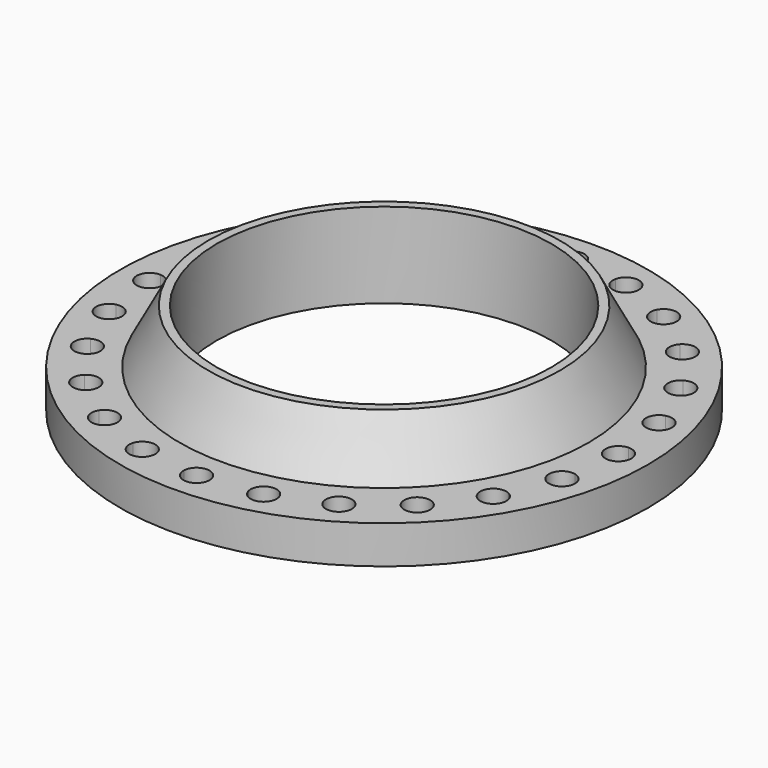
from build123d import *

# Parameters (mm, degrees)
F0_R     = 45.75
F0_R_2   = 35.5
F0_R_3   = 29
F1_DEPTH = 6.6
F3_DEPTH = 16
F5_R     = 34.75
F6_DEPTH = 1.25


# Not quite as in the source:
# - a fillet or chamfer that OpenCascade refuses, or shapes differently, is made with other operations: its cross-section is extruded or revolved along the edge and cut away or added
# - the program builds the solid bodies; features that only make, move or delete a surface that nothing else refers to are left out


with BuildPart() as f1:
    # F0 (on Top) → F1 (new body)
    with BuildSketch(Plane.XY):
        Circle(F0_R)
        with BuildLine():
            ThreePointArc((39.7626716036, 8.3258976659), (40.2774474933, 5.3026265589), (40.5626923077, 2.2491371126))
            ThreePointArc((40.5626923077, 2.2491371126), (42.1938065037, 1.6128689202), (42.875, 0))
            ThreePointArc((42.875, 0), (42.1938065037, -1.6128689202), (40.5626923077, -2.2491371126))
            ThreePointArc((40.5626923077, -2.2491371126), (40.2774474933, -5.3026265589), (39.7626716036, -8.3258976659))
            ThreePointArc((39.7626716036, -8.3258976659), (41.0066434783, -9.1202234435), (41.490736693, -10.5145237073))
            ThreePointArc((41.490736693, -10.5145237073), (40.5856002009, -12.3183646496), (38.598432564, -12.6708969138))
            ThreePointArc((38.598432564, -12.6708969138), (37.5326060083, -15.5465144398), (36.2528905407, -18.3335362777))
            ThreePointArc((36.2528905407, -18.3335362777), (37.115073941, -19.1606252568), (37.4322820287, -20.3125))
            ThreePointArc((37.4322820287, -20.3125), (36.2801915533, -22.2764487457), (34.003753428, -22.22915603))
            ThreePointArc((34.003753428, -22.22915603), (32.2299794493, -24.7309330535), (30.2725348981, -27.0917746898))
            ThreePointArc((30.2725348981, -27.0917746898), (30.7928194193, -27.8364726592), (30.9762129857, -28.7262129857))
            ThreePointArc((30.9762129857, -28.7262129857), (29.5583829906, -30.8166658273), (27.0917746898, -30.2725348981))
            ThreePointArc((27.0917746898, -30.2725348981), (24.7309330535, -32.2299794493), (22.22915603, -34.003753428))
            ThreePointArc((22.22915603, -34.003753428), (22.477560746, -34.5698998227), (22.5625, -35.1822820287))
            ThreePointArc((22.5625, -35.1822820287), (20.8646918257, -37.3634707385), (18.3335362777, -36.2528905407))
            ThreePointArc((18.3335362777, -36.2528905407), (15.5465144398, -37.5326060083), (12.6708969138, -38.598432564))
            ThreePointArc((12.6708969138, -38.598432564), (12.740993976, -38.9161906367), (12.7645237073, -39.240736693))
            ThreePointArc((12.7645237073, -39.240736693), (10.7772891986, -41.4753405274), (8.3258976659, -39.7626716036))
            ThreePointArc((8.3258976659, -39.7626716036), (5.3026265589, -40.2774474933), (2.2491371126, -40.5626923077))
            ThreePointArc((2.2491371126, -40.5626923077), (2.2497842678, -40.5938431665), (2.25, -40.625))
            ThreePointArc((2.25, -40.625), (-0.0311568335, -42.8747842678), (-2.2491371126, -40.5626923077))
            ThreePointArc((-2.2491371126, -40.5626923077), (-5.3026265589, -40.2774474933), (-8.3258976659, -39.7626716036))
            ThreePointArc((-8.3258976659, -39.7626716036), (-11.0968665588, -41.4140698021), (-12.6708969138, -38.598432564))
            ThreePointArc((-12.6708969138, -38.598432564), (-15.5465144398, -37.5326060083), (-18.3335362777, -36.2528905407))
            ThreePointArc((-18.3335362777, -36.2528905407), (-21.4375, -37.1308391873), (-22.22915603, -34.003753428))
            ThreePointArc((-22.22915603, -34.003753428), (-24.7309330535, -32.2299794493), (-27.0917746898, -30.2725348981))
            ThreePointArc((-27.0917746898, -30.2725348981), (-30.3172032434, -30.3172032434), (-30.2725348981, -27.0917746898))
            ThreePointArc((-30.2725348981, -27.0917746898), (-32.2299794493, -24.7309330535), (-34.003753428, -22.22915603))
            ThreePointArc((-34.003753428, -22.22915603), (-37.1308391873, -21.4375), (-36.2528905407, -18.3335362777))
            ThreePointArc((-36.2528905407, -18.3335362777), (-37.5326060083, -15.5465144398), (-38.598432564, -12.6708969138))
            ThreePointArc((-38.598432564, -12.6708969138), (-41.4140698021, -11.0968665588), (-39.7626716036, -8.3258976659))
            ThreePointArc((-39.7626716036, -8.3258976659), (-40.2774474933, -5.3026265589), (-40.5626923077, -2.2491371126))
            ThreePointArc((-40.5626923077, -2.2491371126), (-42.875, 0), (-40.5626923077, 2.2491371126))
            ThreePointArc((-40.5626923077, 2.2491371126), (-40.2774474933, 5.3026265589), (-39.7626716036, 8.3258976659))
            ThreePointArc((-39.7626716036, 8.3258976659), (-41.4140698021, 11.0968665588), (-38.598432564, 12.6708969138))
            ThreePointArc((-38.598432564, 12.6708969138), (-37.5326060083, 15.5465144398), (-36.2528905407, 18.3335362777))
            ThreePointArc((-36.2528905407, 18.3335362777), (-37.1308391873, 21.4375), (-34.003753428, 22.22915603))
            ThreePointArc((-34.003753428, 22.22915603), (-32.2299794493, 24.7309330535), (-30.2725348981, 27.0917746898))
            ThreePointArc((-30.2725348981, 27.0917746898), (-30.3172032434, 30.3172032434), (-27.0917746898, 30.2725348981))
            ThreePointArc((-27.0917746898, 30.2725348981), (-24.7309330535, 32.2299794493), (-22.22915603, 34.003753428))
            ThreePointArc((-22.22915603, 34.003753428), (-21.4375, 37.1308391873), (-18.3335362777, 36.2528905407))
            ThreePointArc((-18.3335362777, 36.2528905407), (-15.5465144398, 37.5326060083), (-12.6708969138, 38.598432564))
            ThreePointArc((-12.6708969138, 38.598432564), (-11.0968665588, 41.4140698021), (-8.3258976659, 39.7626716036))
            ThreePointArc((-8.3258976659, 39.7626716036), (-5.3026265589, 40.2774474933), (-2.2491371126, 40.5626923077))
            ThreePointArc((-2.2491371126, 40.5626923077), (-0.0311568335, 42.8747842678), (2.25, 40.625))
            ThreePointArc((2.25, 40.625), (2.2497842678, 40.5938431665), (2.2491371126, 40.5626923077))
            ThreePointArc((2.2491371126, 40.5626923077), (5.3026265589, 40.2774474933), (8.3258976659, 39.7626716036))
            ThreePointArc((8.3258976659, 39.7626716036), (10.7772891986, 41.4753405274), (12.7645237073, 39.240736693))
            ThreePointArc((12.7645237073, 39.240736693), (12.740993976, 38.9161906367), (12.6708969138, 38.598432564))
            ThreePointArc((12.6708969138, 38.598432564), (15.5465144398, 37.5326060083), (18.3335362777, 36.2528905407))
            ThreePointArc((18.3335362777, 36.2528905407), (20.8646918257, 37.3634707385), (22.5625, 35.1822820287))
            ThreePointArc((22.5625, 35.1822820287), (22.477560746, 34.5698998227), (22.22915603, 34.003753428))
            ThreePointArc((22.22915603, 34.003753428), (24.7309330535, 32.2299794493), (27.0917746898, 30.2725348981))
            ThreePointArc((27.0917746898, 30.2725348981), (29.5583829906, 30.8166658273), (30.9762129857, 28.7262129857))
            ThreePointArc((30.9762129857, 28.7262129857), (30.7928194193, 27.8364726592), (30.2725348981, 27.0917746898))
            ThreePointArc((30.2725348981, 27.0917746898), (32.2299794493, 24.7309330535), (34.003753428, 22.22915603))
            ThreePointArc((34.003753428, 22.22915603), (36.2801915533, 22.2764487457), (37.4322820287, 20.3125))
            ThreePointArc((37.4322820287, 20.3125), (37.115073941, 19.1606252568), (36.2528905407, 18.3335362777))
            ThreePointArc((36.2528905407, 18.3335362777), (37.5326060083, 15.5465144398), (38.598432564, 12.6708969138))
            ThreePointArc((38.598432564, 12.6708969138), (40.5856002009, 12.3183646496), (41.490736693, 10.5145237073))
            ThreePointArc((41.490736693, 10.5145237073), (41.0066434783, 9.1202234435), (39.7626716036, 8.3258976659))
        make_face(mode=Mode.SUBTRACT)
        with BuildLine():
            ThreePointArc((40.5626923077, -2.2491371126), (38.375, 0), (40.5626923077, 2.2491371126))
            ThreePointArc((40.5626923077, 2.2491371126), (40.2774474933, 5.3026265589), (39.7626716036, 8.3258976659))
            ThreePointArc((39.7626716036, 8.3258976659), (37.0674035838, 9.9321808558), (38.598432564, 12.6708969138))
            ThreePointArc((38.598432564, 12.6708969138), (37.5326060083, 15.5465144398), (36.2528905407, 18.3335362777))
            ThreePointArc((36.2528905407, 18.3335362777), (33.2337248702, 19.1875), (34.003753428, 22.22915603))
            ThreePointArc((34.003753428, 22.22915603), (32.2299794493, 24.7309330535), (30.2725348981, 27.0917746898))
            ThreePointArc((30.2725348981, 27.0917746898), (27.135222728, 27.135222728), (27.0917746898, 30.2725348981))
            ThreePointArc((27.0917746898, 30.2725348981), (24.7309330535, 32.2299794493), (22.22915603, 34.003753428))
            ThreePointArc((22.22915603, 34.003753428), (19.1875, 33.2337248702), (18.3335362777, 36.2528905407))
            ThreePointArc((18.3335362777, 36.2528905407), (15.5465144398, 37.5326060083), (12.6708969138, 38.598432564))
            ThreePointArc((12.6708969138, 38.598432564), (9.9321808558, 37.0674035838), (8.3258976659, 39.7626716036))
            ThreePointArc((8.3258976659, 39.7626716036), (5.3026265589, 40.2774474933), (2.2491371126, 40.5626923077))
            ThreePointArc((2.2491371126, 40.5626923077), (0, 38.375), (-2.2491371126, 40.5626923077))
            ThreePointArc((-2.2491371126, 40.5626923077), (-5.3026265589, 40.2774474933), (-8.3258976659, 39.7626716036))
            ThreePointArc((-8.3258976659, 39.7626716036), (-8.2799198729, 39.5035021843), (-8.2645237073, 39.240736693))
            ThreePointArc((-8.2645237073, 39.240736693), (-10.189977651, 37.0142664243), (-12.6708969138, 38.598432564))
            ThreePointArc((-12.6708969138, 38.598432564), (-15.5465144398, 37.5326060083), (-18.3335362777, 36.2528905407))
            ThreePointArc((-18.3335362777, 36.2528905407), (-18.1313112902, 35.7344738545), (-18.0625, 35.1822820287))
            ThreePointArc((-18.0625, 35.1822820287), (-19.700117794, 33.0172212828), (-22.22915603, 34.003753428))
            ThreePointArc((-22.22915603, 34.003753428), (-24.7309330535, 32.2299794493), (-27.0917746898, 30.2725348981))
            ThreePointArc((-27.0917746898, 30.2725348981), (-26.6357601441, 29.5583829906), (-26.4762129857, 28.7262129857))
            ThreePointArc((-26.4762129857, 28.7262129857), (-27.8364726592, 26.6596065521), (-30.2725348981, 27.0917746898))
            ThreePointArc((-30.2725348981, 27.0917746898), (-32.2299794493, 24.7309330535), (-34.003753428, 22.22915603))
            ThreePointArc((-34.003753428, 22.22915603), (-33.218333283, 21.4104095246), (-32.9322820287, 20.3125))
            ThreePointArc((-32.9322820287, 20.3125), (-34.0304072855, 18.3797080878), (-36.2528905407, 18.3335362777))
            ThreePointArc((-36.2528905407, 18.3335362777), (-37.5326060083, 15.5465144398), (-38.598432564, 12.6708969138))
            ThreePointArc((-38.598432564, 12.6708969138), (-37.4368957507, 11.8593872152), (-36.990736693, 10.5145237073))
            ThreePointArc((-36.990736693, 10.5145237073), (-37.8464364292, 8.748616922), (-39.7626716036, 8.3258976659))
            ThreePointArc((-39.7626716036, 8.3258976659), (-40.2774474933, 5.3026265589), (-40.5626923077, 2.2491371126))
            ThreePointArc((-40.5626923077, 2.2491371126), (-39.0121310798, 1.5688065037), (-38.375, 0))
            ThreePointArc((-38.375, 0), (-39.0121310798, -1.5688065037), (-40.5626923077, -2.2491371126))
            ThreePointArc((-40.5626923077, -2.2491371126), (-40.2774474933, -5.3026265589), (-39.7626716036, -8.3258976659))
            ThreePointArc((-39.7626716036, -8.3258976659), (-37.8464364292, -8.748616922), (-36.990736693, -10.5145237073))
            ThreePointArc((-36.990736693, -10.5145237073), (-37.4368957507, -11.8593872152), (-38.598432564, -12.6708969138))
            ThreePointArc((-38.598432564, -12.6708969138), (-37.5326060083, -15.5465144398), (-36.2528905407, -18.3335362777))
            ThreePointArc((-36.2528905407, -18.3335362777), (-34.0304072855, -18.3797080878), (-32.9322820287, -20.3125))
            ThreePointArc((-32.9322820287, -20.3125), (-33.218333283, -21.4104095246), (-34.003753428, -22.22915603))
            ThreePointArc((-34.003753428, -22.22915603), (-32.2299794493, -24.7309330535), (-30.2725348981, -27.0917746898))
            ThreePointArc((-30.2725348981, -27.0917746898), (-27.8364726592, -26.6596065521), (-26.4762129857, -28.7262129857))
            ThreePointArc((-26.4762129857, -28.7262129857), (-26.6357601441, -29.5583829906), (-27.0917746898, -30.2725348981))
            ThreePointArc((-27.0917746898, -30.2725348981), (-24.7309330535, -32.2299794493), (-22.22915603, -34.003753428))
            ThreePointArc((-22.22915603, -34.003753428), (-19.700117794, -33.0172212828), (-18.0625, -35.1822820287))
            ThreePointArc((-18.0625, -35.1822820287), (-18.1313112902, -35.7344738545), (-18.3335362777, -36.2528905407))
            ThreePointArc((-18.3335362777, -36.2528905407), (-15.5465144398, -37.5326060083), (-12.6708969138, -38.598432564))
            ThreePointArc((-12.6708969138, -38.598432564), (-10.189977651, -37.0142664243), (-8.2645237073, -39.240736693))
            ThreePointArc((-8.2645237073, -39.240736693), (-8.2799198729, -39.5035021843), (-8.3258976659, -39.7626716036))
            ThreePointArc((-8.3258976659, -39.7626716036), (-5.3026265589, -40.2774474933), (-2.2491371126, -40.5626923077))
            ThreePointArc((-2.2491371126, -40.5626923077), (0, -38.375), (2.2491371126, -40.5626923077))
            ThreePointArc((2.2491371126, -40.5626923077), (5.3026265589, -40.2774474933), (8.3258976659, -39.7626716036))
            ThreePointArc((8.3258976659, -39.7626716036), (9.9321808558, -37.0674035838), (12.6708969138, -38.598432564))
            ThreePointArc((12.6708969138, -38.598432564), (15.5465144398, -37.5326060083), (18.3335362777, -36.2528905407))
            ThreePointArc((18.3335362777, -36.2528905407), (19.1875, -33.2337248702), (22.22915603, -34.003753428))
            ThreePointArc((22.22915603, -34.003753428), (24.7309330535, -32.2299794493), (27.0917746898, -30.2725348981))
            ThreePointArc((27.0917746898, -30.2725348981), (27.135222728, -27.135222728), (30.2725348981, -27.0917746898))
            ThreePointArc((30.2725348981, -27.0917746898), (32.2299794493, -24.7309330535), (34.003753428, -22.22915603))
            ThreePointArc((34.003753428, -22.22915603), (33.2337248702, -19.1875), (36.2528905407, -18.3335362777))
            ThreePointArc((36.2528905407, -18.3335362777), (37.5326060083, -15.5465144398), (38.598432564, -12.6708969138))
            ThreePointArc((38.598432564, -12.6708969138), (37.0674035838, -9.9321808558), (39.7626716036, -8.3258976659))
            ThreePointArc((39.7626716036, -8.3258976659), (40.2774474933, -5.3026265589), (40.5626923077, -2.2491371126))
        make_face()
        Circle(F0_R_2, mode=Mode.SUBTRACT)
        Circle(F0_R_2)
        Circle(F0_R_3, mode=Mode.SUBTRACT)
    extrude(amount=F1_DEPTH)

    # F0 (on Top) → F3 (join)
    with BuildSketch(Plane.XY):
        Circle(F0_R_2)
        Circle(F0_R_3, mode=Mode.SUBTRACT)
    extrude(amount=F3_DEPTH)

    # F4: chamfer of 5 x 9.5 on 1 edges, made by hand


with BuildPart() as f4_tool2:
    # F4_s3 → F4_t4 (revolve)
    with BuildSketch(Plane.XZ):
        Polygon((35.5, 6.5), (30.5, 16), (35.5, 16), align=None)
    revolve(axis=Axis((0, 0, 16), (0, 0, 1)))

    split(bisect_by=Plane.XY.offset(6.6), keep=Keep.TOP)


with BuildPart() as f1_1:
    add(f1.part)

    # F4_t1: cut F4_tool2
    add(f4_tool2.part, mode=Mode.SUBTRACT)

    # F5 (on Top) → F6 (cut)
    with BuildSketch(Plane.XY):
        Circle(F5_R)
    extrude(amount=F6_DEPTH, mode=Mode.SUBTRACT)


solid = f1_1.part
